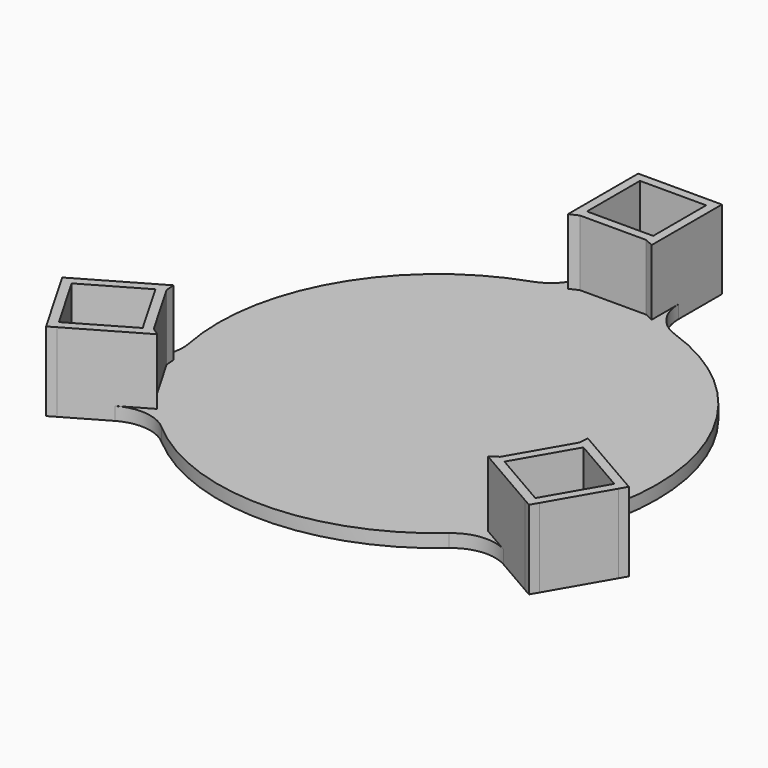
from build123d import *

# Parameters (mm, degrees)
F0_R     = 50
F1_DEPTH = 3
F2_W     = 15.1
F2_H     = 15.1
F3_DEPTH = 3
F2_H_2   = 2
F2_W_2   = 2
F4_DEPTH = 18
F5_R     = 10


with BuildPart() as f1:
    # F0 (on Top) → F1 (new body)
    with BuildSketch(Plane.XY):
        Circle(F0_R)
    extrude(amount=F1_DEPTH)

    # F2 (on Top) → F3, piece 3 (join)
    with BuildSketch(Plane.XY):
        with BuildLine():
            ThreePointArc((-9.55, 49.0795018312), (-4.7971297897, 49.7693434333), (0, 50))
            Line((0, 50), (-7.55, 50))
            Line((-7.55, 50), (-9.55, 49.0795018312))
        make_face()
        with BuildLine():
            ThreePointArc((0, 50), (4.7971297897, 49.7693434333), (9.55, 49.0795018312))
            Line((9.55, 49.0795018312), (7.55, 50))
            Line((7.55, 50), (0, 50))
        make_face()
        with BuildLine():
            Line((47.0762701892, -18.4615082014), (47.2790953909, -16.2692083095))
            ThreePointArc((47.2790953909, -16.2692083095), (45.5000807553, -20.7302351954), (43.3012704728, -24.9999995088))
            Line((43.3012704728, -24.9999995088), (47.0762701892, -18.4615082014))
        make_face()
        with BuildLine():
            Line((39.5262701892, -31.5384917986), (43.3012704728, -24.9999995088))
            ThreePointArc((43.3012704728, -24.9999995088), (40.7029510127, -29.039107749), (37.7290953909, -32.8102935217))
            Line((37.7290953909, -32.8102935217), (39.5262701892, -31.5384917986))
        make_face()
        with BuildLine():
            ThreePointArc((-43.3012707255, -24.9999990711), (-45.5000808601, -20.7302349654), (-47.2790953909, -16.2692083095))
            Line((-47.2790953909, -16.2692083095), (-47.0762701892, -18.4615082014))
            Line((-47.0762701892, -18.4615082014), (-43.3012707255, -24.9999990711))
        make_face()
        with BuildLine():
            Line((-39.5262701892, -31.5384917986), (-37.7290953909, -32.8102935217))
            ThreePointArc((-37.7290953909, -32.8102935217), (-40.7029511595, -29.0391075432), (-43.3012707255, -24.9999990711))
            Line((-43.3012707255, -24.9999990711), (-39.5262701892, -31.5384917986))
        make_face()
    extrude(amount=F3_DEPTH)



with BuildPart() as f3:
    # F2 (on Top) → F3 (new body)
    with BuildSketch(Plane.XY):
        with Locations((0, 59.55)):
            Rectangle(F2_W, F2_H)
    extrude(amount=F3_DEPTH)


with BuildPart() as f3b:
    # F2 (on Top) → F3, piece 2 (new body)
    with BuildSketch(Plane.XY):
        Polygon((54.3353045939, -40.0884917986), (61.8853045939, -27.0115082014), (48.8083209968, -19.4615082014), (41.2583209968, -32.5384917986), align=None)
    extrude(amount=F3_DEPTH)


with BuildPart() as f3c:
    # F2 (on Top) → F3, piece 4 (new body)
    with BuildSketch(Plane.XY):
        Polygon((-48.8083209968, -19.4615082014), (-61.8853045939, -27.0115082014), (-54.3353045939, -40.0884917986), (-41.2583209968, -32.5384917986), align=None)
    extrude(amount=F3_DEPTH)


with BuildPart() as f1_1:
    add(f1.part)

    add(f3.part)  # F4 merges F3

    add(f3b.part)  # F4 merges F3b

    add(f3c.part)  # F4 merges F3c
    # F2 (on Top) → F4 (join)
    with BuildSketch(Plane.XY):
        Polygon((-47.0762701892, -18.4615082014), (-47.2790953909, -16.2692083095), (-62.8853045939, -25.2794573939), (-61.8853045939, -27.0115082014), (-48.8083209968, -19.4615082014), align=None)
        Polygon((-39.5262701892, -31.5384917986), (-43.3012707255, -24.9999990711), (-47.0762701892, -18.4615082014), (-48.8083209968, -19.4615082014), (-41.2583209968, -32.5384917986), align=None)
        Polygon((-53.3353045939, -41.8205426061), (-37.7290953909, -32.8102935217), (-39.5262701892, -31.5384917986), (-41.2583209968, -32.5384917986), (-54.3353045939, -40.0884917986), align=None)
        Polygon((-54.3353045939, -40.0884917986), (-61.8853045939, -27.0115082014), (-63.6173554015, -28.0115082014), (-56.0673554015, -41.0884917986), align=None)
        Polygon((-61.8853045939, -27.0115082014), (-62.8853045939, -25.2794573939), (-64.6173554015, -26.2794573939), (-63.6173554015, -28.0115082014), align=None)
        Polygon((-55.0673554015, -42.8205426061), (-53.3353045939, -41.8205426061), (-54.3353045939, -40.0884917986), (-56.0673554015, -41.0884917986), align=None)
        Polygon((47.0762701892, -18.4615082014), (43.3012704728, -24.9999995088), (39.5262701892, -31.5384917986), (41.2583209968, -32.5384917986), (48.8083209968, -19.4615082014), align=None)
        Polygon((62.8853045939, -25.2794573939), (47.2790953909, -16.2692083095), (47.0762701892, -18.4615082014), (48.8083209968, -19.4615082014), (61.8853045939, -27.0115082014), align=None)
        Polygon((64.6173554015, -26.2794573939), (62.8853045939, -25.2794573939), (61.8853045939, -27.0115082014), (63.6173554015, -28.0115082014), align=None)
        Polygon((63.6173554015, -28.0115082014), (61.8853045939, -27.0115082014), (54.3353045939, -40.0884917986), (56.0673554015, -41.0884917986), align=None)
        Polygon((54.3353045939, -40.0884917986), (53.3353045939, -41.8205426061), (55.0673554015, -42.8205426061), (56.0673554015, -41.0884917986), align=None)
        Polygon((39.5262701892, -31.5384917986), (37.7290953909, -32.8102935217), (53.3353045939, -41.8205426061), (54.3353045939, -40.0884917986), (41.2583209968, -32.5384917986), align=None)
        with Locations((0, 68.1)):
            Rectangle(F2_W, F2_H_2)
        with Locations((-8.55, 68.1)):
            Rectangle(F2_W_2, F2_H_2)
        with Locations((8.55, 68.1)):
            Rectangle(F2_W_2, F2_H_2)
        Polygon((7.55, 50), (9.55, 49.0795018312), (9.55, 67.1), (7.55, 67.1), (7.55, 52), align=None)
        Polygon((-9.55, 67.1), (-9.55, 49.0795018312), (-7.55, 50), (-7.55, 52), (-7.55, 67.1), align=None)
        Polygon((-7.55, 50), (0, 50), (7.55, 50), (7.55, 52), (-7.55, 52), align=None)
    extrude(amount=F4_DEPTH)

    # F5
    f5_edges = [f1_1.edges().sort_by_distance(p)[0] for p in [
        (-9.55, 49.079502, 1.5),
        (9.55, 49.079502, 1.5),
        (-47.279095, -16.269208, 1.5),
        (-37.729095, -32.810294, 1.5),
        (37.729095, -32.810294, 1.5),
        (47.279095, -16.269208, 1.5),
    ]]
    fillet(f5_edges, radius=F5_R)


solid = f1_1.part
